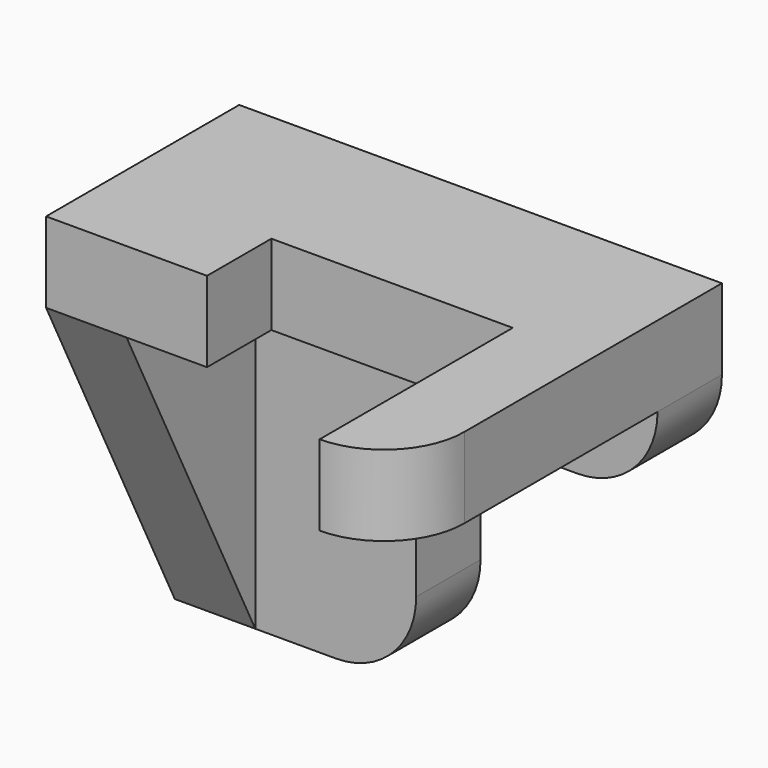
from build123d import *

# Parameters (mm, degrees)
F1_DEPTH  = 1270
F2_W      = 508
F2_H      = 762
F3_DEPTH  = 1016
F4_W      = 1270
F4_H      = 254
F5_DEPTH  = 1016
F6_W      = 762
F6_H      = 762
F7_DEPTH  = 254.001
F8_W      = 508
F8_H      = 1016
F9_DEPTH  = 254.001
F11_DEPTH = 254.001
F12_W     = 508
F12_H     = 508
F13_DEPTH = 254.001
F14_R     = 254
F15_R     = 253.99999


# Not quite as in the source:
# - a fillet or chamfer is up to 0.001 mm smaller than in the source, because OpenCascade refuses the exact size


with BuildPart() as f1:
    # F0 (on Front) → F1 (new body)
    with BuildSketch(Plane.XZ):
        Polygon((0, 1270), (0, 0), (762, 0), (762, 762), (1524, 762), (1524, 1270), align=None)
    extrude(amount=F1_DEPTH)

    # F2 (on face) → F3 (cut)
    with BuildSketch(Plane.XZ.offset(1270)):
        with Locations((508, 381)):
            Rectangle(F2_W, F2_H)
    extrude(amount=-F3_DEPTH, mode=Mode.SUBTRACT)

    # F4 (on face) → F5 (cut)
    with BuildSketch(Plane.XZ.offset(1270)):
        with Locations((889, 889)):
            Rectangle(F4_W, F4_H)
    extrude(amount=-F5_DEPTH, mode=Mode.SUBTRACT)

    # F6 (on face) → F7 (cut, through all)
    with BuildSketch(Plane(origin=(0, 0, 1016), x_dir=(1, 0, 0), z_dir=(0, 0, -1))):
        with Locations((889, 889)):
            Rectangle(F6_W, F6_H)
    extrude(amount=-F7_DEPTH, mode=Mode.SUBTRACT)

    # F8 (on face) → F9 (cut, through all)
    with BuildSketch(Plane.YZ.offset(254)):
        with Locations((-1016, 508)):
            Rectangle(F8_W, F8_H)
    extrude(amount=-F9_DEPTH, mode=Mode.SUBTRACT)

    # F10 (on face) → F11 (cut, through all)
    with BuildSketch(Plane.YZ.offset(254)):
        Polygon((-254, 0), (-762, 1016), (-762, 0), align=None)
    extrude(amount=-F11_DEPTH, mode=Mode.SUBTRACT)

    # F12 (on face) → F13 (cut, through all)
    with BuildSketch(Plane(origin=(0, 0, 1016), x_dir=(1, 0, 0), z_dir=(0, 0, -1))):
        with Locations((254, 1016)):
            Rectangle(F12_W, F12_H)
    extrude(amount=-F13_DEPTH, mode=Mode.SUBTRACT)

    # F14
    f14_edges = [f1.edges().sort_by_distance(p)[0] for p in [
        (762, -127, 0),
        (1524, -127, 762),
    ]]
    fillet(f14_edges, radius=F14_R)

    # F15 (radius 254 in the source; OpenCascade refuses exactly that, so slightly less here)
    f15_edges = [f1.edges().sort_by_distance(p)[0] for p in [
        (1524, -1270, 1143),
    ]]
    fillet(f15_edges, radius=F15_R)


solid = f1.part
